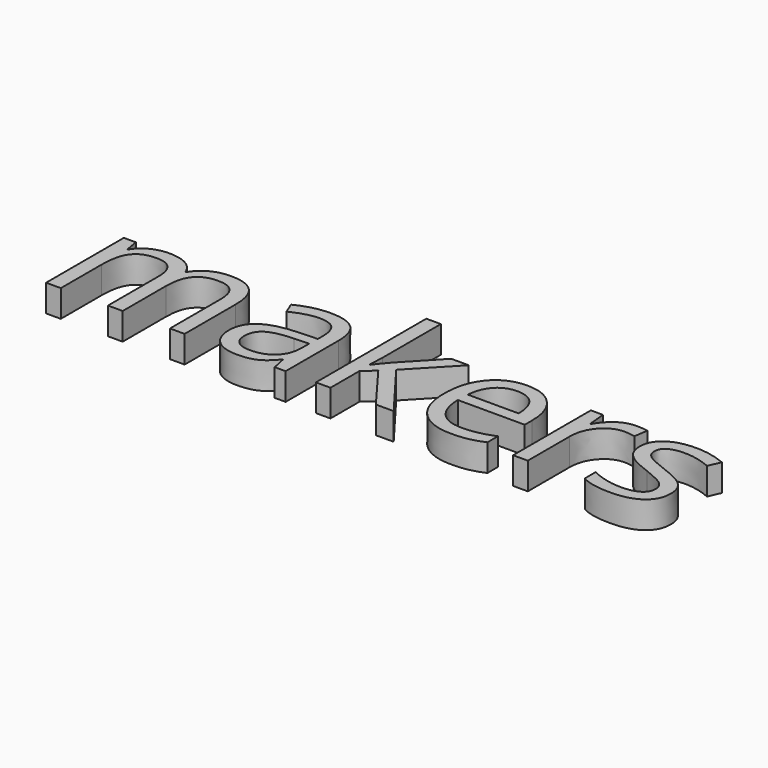
from build123d import *

# Parameters (mm, degrees)
F0_TEXT_SIZE = 33.5671706125
F1_DEPTH     = 5


# Not quite as in the source:
# - Text() gives the source's letters only with a copy of the font that has no kerning and outlines rounded to 1/6400 em; it was checked with that copy


with BuildPart() as f1:
    # F0 (on Top) → F1 (new body)
    with BuildSketch(Plane.XY):
        with Locations((0, 0)):
            Text('makers', F0_TEXT_SIZE, font='Open Sans', text_align=(TextAlign.LEFT, TextAlign.BOTTOM))
    extrude(amount=F1_DEPTH)


solid = f1.part
